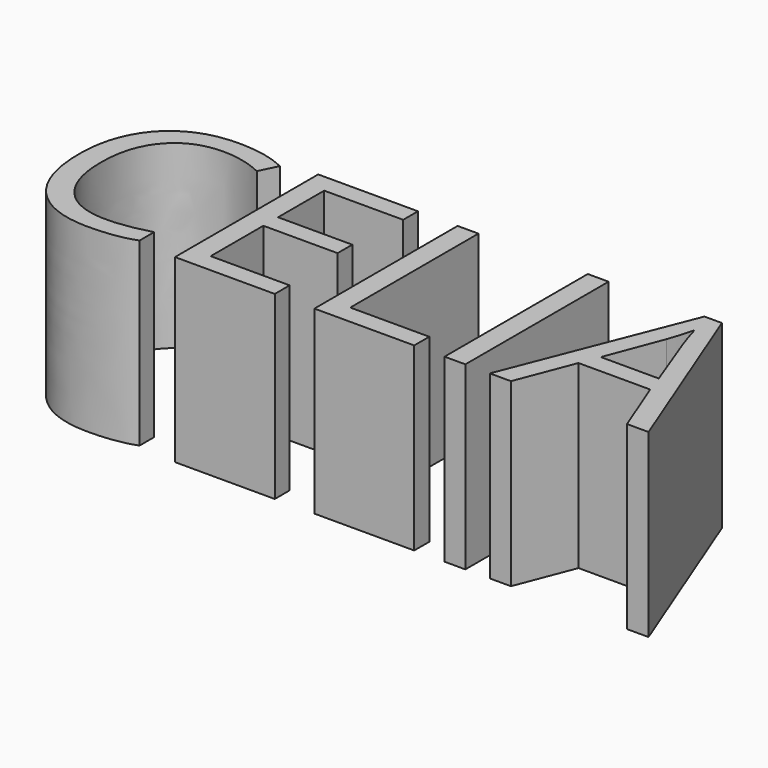
from build123d import *

# Parameters (mm, degrees)
F0_TEXT_SIZE = 35.2777777778
F1_DEPTH     = 25.4


# Not quite as in the source:
# - Text() gives the source's letters only with a copy of the font that has no kerning and outlines rounded to 1/6400 em; it was checked with that copy


with BuildPart() as f1:
    # F0 (on Top) → F1 (new body)
    with BuildSketch(Plane.XY):
        with Locations((-24.2810574305, -8.2801761229)):
            Text('CELIA', F0_TEXT_SIZE, font='Open Sans', text_align=(TextAlign.LEFT, TextAlign.BOTTOM))
    extrude(amount=F1_DEPTH)


solid = f1.part
